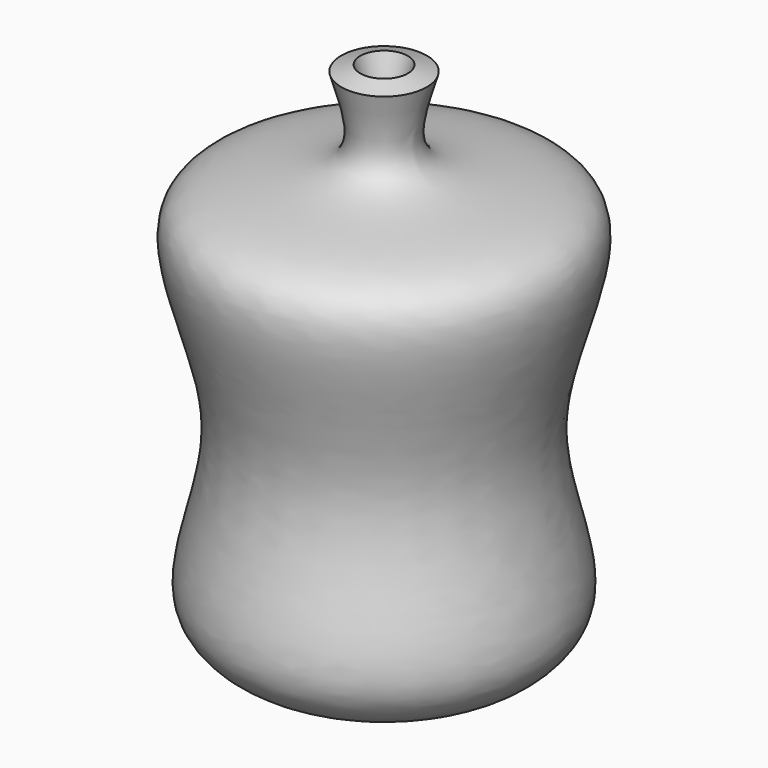
from build123d import *


# Not quite as in the source:
# - the dataset's text gives a spline's control points without its knots; the knots are read off the source's solid
# - the program builds the solid bodies; features that only make, move or delete a surface that nothing else refers to are left out


with BuildPart() as f1:
    # F0 (on Front) → F1 (revolve)
    with BuildSketch(Plane.XZ):
        with BuildLine():
            Line((1.1614379512, 2.2589072326), (0, 0))
            add(Edge.make_bspline(
                [(0, 0), (3.8459840264, -1.9774480969), (11.3490841659, -5.8352361141), (25.5374042238, 2.6183556947), (12.973930999, 23.2300931111), (30.3859263682, 52.1179596023), (2.3575024196, 49.6014051841), (4.4064391538, 59.1449342316), (5.1489751192, 61.5357891641), (5.4707699455, 62.5719204545)],
                knots=[0, 0, 0, 0, 0.1409162059, 0.2749123234, 0.4596152363, 0.6554531535, 0.8210686524, 0.9224560363, 1, 1, 1, 1], degree=3))
            Line((5.4707699455, 62.5719204545), (3.0450640502, 63.3252802021))
            add(Edge.make_bspline(
                [(1.1614379512, 2.2589072326), (2.0143348912, 1.8203824183), (3.6830048523, 0.9629966166), (6.0810150463, -0.1160701228), (7.9803648698, -0.7337995168), (9.4367571204, -1.0133945472), (10.3243895837, -1.0931634434), (11.0270661777, -1.0963468471), (11.5509810389, -1.0674450968), (12.0807205793, -1.0051409907), (12.7987526582, -0.8767074007), (13.6999523681, -0.632880996), (14.7475772611, -0.2156840882), (15.7218903939, 0.3121102466), (16.5872285703, 0.9319532963), (17.3134057846, 1.6213112478), (17.8793478265, 2.3554775234), (18.2115061687, 2.9898201336), (18.3945795418, 3.5076590896), (18.5264179867, 4.0467716472), (18.6125879537, 4.8508378572), (18.568849843, 6.022620498), (18.3806590939, 7.3862779862), (17.9655216294, 9.4255655359), (17.2192557758, 12.3348621876), (16.4355769846, 15.6391035928), (15.9635781424, 18.4960309929), (15.7343087809, 20.7417791721), (15.6871555852, 22.6903796314), (15.7617341821, 24.2983098079), (15.9151084327, 25.9075229827), (16.2305863321, 27.8990766949), (16.7502763854, 30.250073243), (17.3577879151, 32.5456100877), (18.0027505916, 34.7675734125), (18.6360371522, 36.8934418553), (19.2093927299, 38.8961854195), (19.675827345, 40.7425297176), (19.9916990938, 42.3897939537), (20.1232201382, 43.7822720101), (20.0725867412, 44.6697666013), (19.961873283, 45.1898592371), (19.8561587897, 45.489633404), (19.7571785061, 45.6774698476), (19.6688930503, 45.8062567752), (19.5978465829, 45.8938553926), (19.50849415, 45.9874415278), (19.3571287779, 46.1235095161), (19.102888932, 46.3101250605), (18.6872281923, 46.5461285177), (17.9939288886, 46.8586840439), (16.8946328394, 47.221238747), (15.308323662, 47.5870429618), (13.5509465373, 47.8981085961), (11.7045654171, 48.1837638366), (9.8391825722, 48.4817769164), (8.0114019855, 48.8381039672), (6.5508778514, 49.2331406953), (5.4249692047, 49.6607045281), (4.7382253724, 49.9939812389), (4.2016506192, 50.3164637689), (3.8064620072, 50.5922685625), (3.4262809307, 50.9050067854), (2.9643472861, 51.3535270451), (2.4696474782, 51.9706630475), (1.8720451352, 53.0289974443), (1.4722715819, 54.3865094306), (1.3725938884, 55.9054888466), (1.4893130563, 57.2891346695), (1.6798276316, 58.3225996601), (1.8487767857, 59.0664013395), (1.9741352919, 59.5738366652), (2.0920884459, 60.0355614951), (2.2465061465, 60.6215055803), (2.4318702911, 61.2921927287), (2.7156826924, 62.2649919366), (2.9153816372, 62.9077221965), (3.0450640502, 63.3252802021)],
                knots=[5e-10, 5e-10, 5e-10, 5e-10, 0.0312500005, 0.0625000005, 0.0937500005, 0.1093750005, 0.1250000005, 0.1328125005, 0.1406250005, 0.1484375005, 0.1562500005, 0.1718750005, 0.1875000004, 0.2031250004, 0.2187500004, 0.2343750004, 0.2500000004, 0.2656250004, 0.2734375004, 0.2812500004, 0.2968750004, 0.3125000004, 0.3281250004, 0.3437500004, 0.3750000004, 0.4062500004, 0.4218750004, 0.4375000004, 0.4531250004, 0.4609375004, 0.4687500004, 0.4843750004, 0.5000000004, 0.5156250004, 0.5312500004, 0.5468750004, 0.5625000004, 0.5781250004, 0.5937500004, 0.6093750004, 0.6250000004, 0.6328125004, 0.6406250004, 0.6484375004, 0.6523437504, 0.6562500004, 0.6601562504, 0.6640625004, 0.6718750004, 0.6796875004, 0.6875000004, 0.7031250004, 0.7187500004, 0.7343750004, 0.7500000004, 0.7656250004, 0.7812500004, 0.7968750004, 0.8046875004, 0.8125000004, 0.8164062504, 0.8203125004, 0.8242187504, 0.8281250004, 0.8359375004, 0.8437500004, 0.8593750004, 0.8750000004, 0.8906250004, 0.9062500004, 0.9140625004, 0.9218750004, 0.9296875004, 0.9375000004, 0.9531250004, 0.9687500004, 1.0000000004, 1.0000000004, 1.0000000004, 1.0000000004], degree=3))
        make_face()
        Polygon((0, 6.4965388738), (0, 0), (1.1614379512, 2.2589072326), align=None)
    revolve(axis=Axis((0, 0, 3.2482694369), (0, 0, 1)))


solid = f1.part
